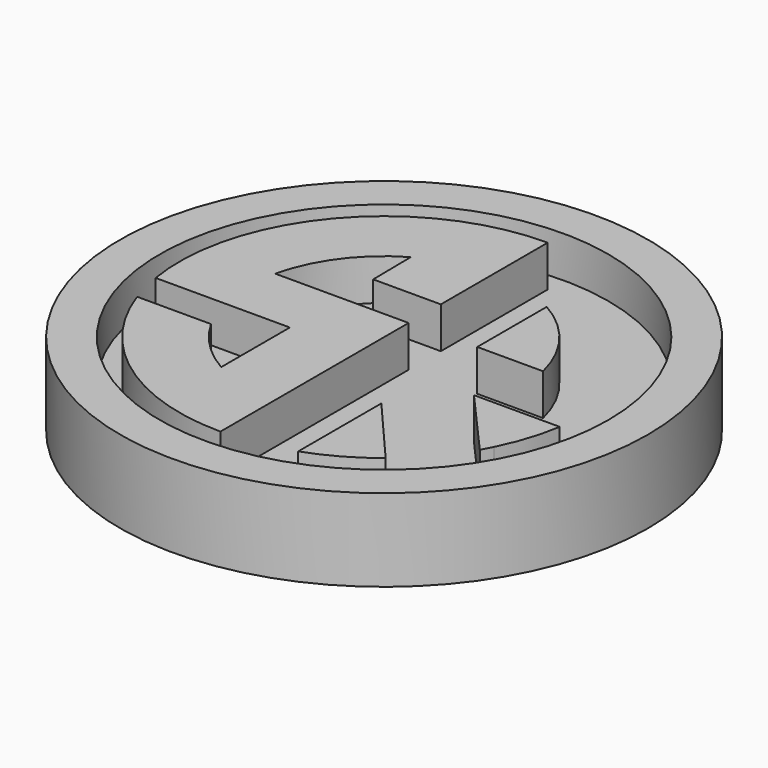
from build123d import *

# Parameters (mm, degrees)
F0_R     = 34.544
F1_DEPTH = 6.35
F0_R_2   = 40.64
F2_DEPTH = 12.7


with BuildPart() as f1:
    # F0 (on Top) → F1 (new body)
    with BuildSketch(Plane.XY):
        Circle(F0_R)
        with BuildLine():
            ThreePointArc((-31.076682867, -5.1222844495), (-24.0138448298, 20.3797269974), (0, 31.496))
            Line((0, 31.496), (0, 10.922))
            Line((0, 10.922), (-10.414, 10.922))
            Line((-10.414, 10.922), (-10.5108203487, 18.2749385662))
            ThreePointArc((-10.5108203487, 18.2749385662), (-16.9420488689, 12.5466212234), (-20.5458211965, 4.7244))
            Line((-20.5458211965, 4.7244), (0, 4.7244))
            Line((0, 4.7244), (0, -31.496))
            ThreePointArc((0, -31.496), (-18.2512319231, -25.6688634203), (-29.7490715955, -10.3436335592))
            Line((-29.7490715955, -10.3436335592), (-18.3700835271, -10.3436335592))
            ThreePointArc((-18.3700835271, -10.3436335592), (-14.9357796661, -14.8786158552), (-10.414, -18.3302844495))
            Line((-10.414, -18.3302844495), (-10.414, -5.1222844495))
            Line((-10.414, -5.1222844495), (-31.076682867, -5.1222844495))
        make_face(mode=Mode.SUBTRACT)
        with BuildLine():
            ThreePointArc((19.8204750869, -24.4774750195), (15.3939322044, -27.477715831), (10.523637749, -29.6858731475))
            Line((10.523637749, -29.6858731475), (10.523637749, -13.6838731475))
            Line((10.523637749, -13.6838731475), (19.8204750869, -24.4774750195))
        make_face(mode=Mode.SUBTRACT)
        with BuildLine():
            ThreePointArc((31.0882471472, -5.0516240273), (29.9760430145, -9.6661709684), (28.1829993455, -14.0611722091))
            ThreePointArc((28.1829993455, -14.0611722091), (27.753918864, -14.8901982421), (27.3004586922, -15.7061443772))
            Line((27.3004586922, -15.7061443772), (17.8802471472, -5.0516240273))
            Line((17.8802471472, -5.0516240273), (31.0882471472, -5.0516240273))
        make_face(mode=Mode.SUBTRACT)
        with BuildLine():
            ThreePointArc((10.3465438025, 18.3684445543), (16.8012840648, 12.7345034365), (20.4811438025, 4.9973465502))
            Line((20.4811438025, 4.9973465502), (10.3465438025, 4.9973465502))
            Line((10.3465438025, 4.9973465502), (10.3465438025, 18.3684445543))
        make_face(mode=Mode.SUBTRACT)
    extrude(amount=F1_DEPTH)

    # F0 (on Top) → F2 (join)
    with BuildSketch(Plane.XY):
        Circle(F0_R_2)
        Circle(F0_R, mode=Mode.SUBTRACT)
        with BuildLine():
            Line((0, 10.922), (0, 31.496))
            ThreePointArc((0, 31.496), (-24.0138448298, 20.3797269974), (-31.076682867, -5.1222844495))
            Line((-31.076682867, -5.1222844495), (-10.414, -5.1222844495))
            Line((-10.414, -5.1222844495), (-10.414, -18.3302844495))
            ThreePointArc((-10.414, -18.3302844495), (-14.9357796661, -14.8786158552), (-18.3700835271, -10.3436335592))
            Line((-18.3700835271, -10.3436335592), (-29.7490715955, -10.3436335592))
            ThreePointArc((-29.7490715955, -10.3436335592), (-18.2512319231, -25.6688634203), (0, -31.496))
            Line((0, -31.496), (0, 4.7244))
            Line((0, 4.7244), (-20.5458211965, 4.7244))
            ThreePointArc((-20.5458211965, 4.7244), (-16.9420488689, 12.5466212234), (-10.5108203487, 18.2749385662))
            Line((-10.5108203487, 18.2749385662), (-10.414, 10.922))
            Line((-10.414, 10.922), (0, 10.922))
        make_face()
        with BuildLine():
            Line((10.3465438025, 4.9973465502), (20.4811438025, 4.9973465502))
            ThreePointArc((20.4811438025, 4.9973465502), (16.8012840648, 12.7345034365), (10.3465438025, 18.3684445543))
            Line((10.3465438025, 18.3684445543), (10.3465438025, 4.9973465502))
        make_face()
        with BuildLine():
            Line((10.523637749, -13.6838731475), (10.523637749, -29.6858731475))
            ThreePointArc((10.523637749, -29.6858731475), (15.3939322044, -27.477715831), (19.8204750869, -24.4774750195))
            Line((19.8204750869, -24.4774750195), (10.523637749, -13.6838731475))
        make_face()
        with BuildLine():
            ThreePointArc((27.3004586922, -15.7061443772), (27.753918864, -14.8901982421), (28.1829993455, -14.0611722091))
            ThreePointArc((28.1829993455, -14.0611722091), (29.9760430145, -9.6661709684), (31.0882471472, -5.0516240273))
            Line((31.0882471472, -5.0516240273), (17.8802471472, -5.0516240273))
            Line((17.8802471472, -5.0516240273), (27.3004586922, -15.7061443772))
        make_face()
    extrude(amount=F2_DEPTH)


solid = f1.part
